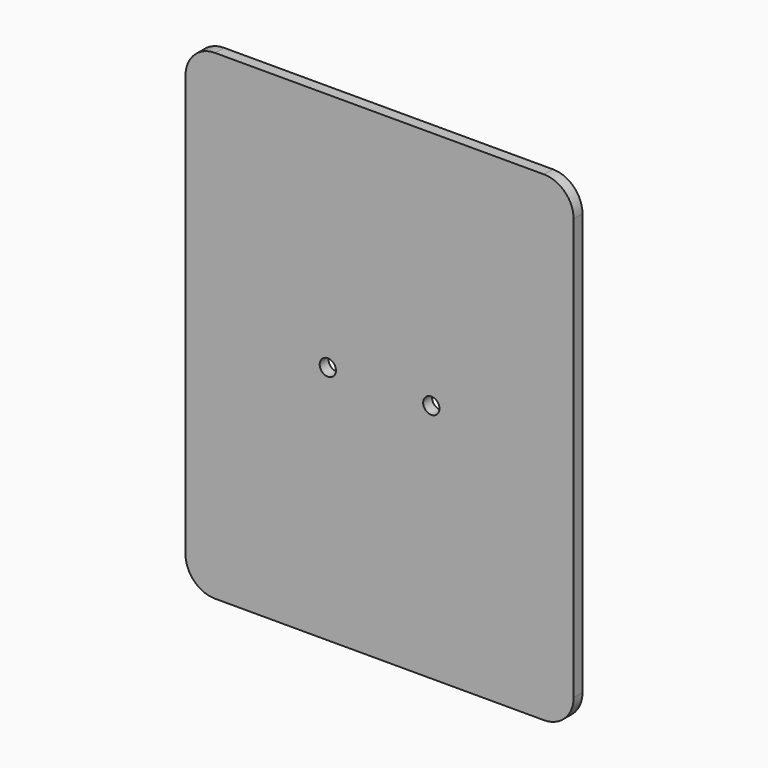
from build123d import *

# Parameters (mm, degrees)
F0_W     = 105
F0_H     = 130
F1_DEPTH = 3
F3_D     = 4.4
F4_R     = 8


with BuildPart() as f1:
    # F0 (on Front) → F1 (new body)
    with BuildSketch(Plane.XZ):
        Rectangle(F0_W, F0_H)
    extrude(amount=F1_DEPTH)

    # F3 (through all)
    with Locations(Plane.XZ.offset(3)):
        with Locations((-14, 0), (14, 0)):
            Hole(F3_D / 2)

    # F4
    f4_edges = [f1.edges().sort_by_distance(p)[0] for p in [
        (52.5, -1.5, 65),
        (-52.5, -1.5, 65),
        (-52.5, -1.5, -65),
        (52.5, -1.5, -65),
    ]]
    fillet(f4_edges, radius=F4_R)


solid = f1.part
